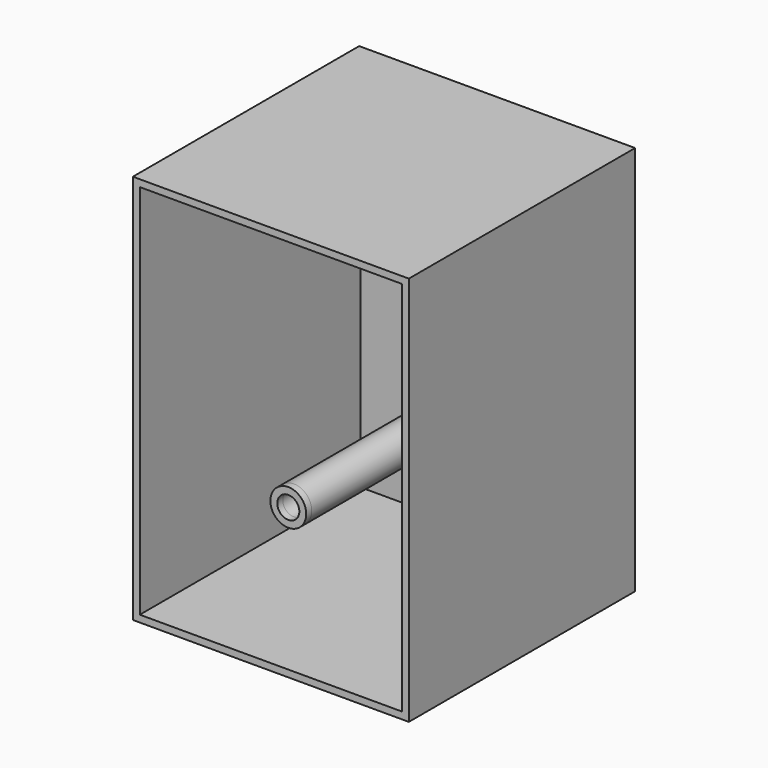
from build123d import *

# Parameters (mm, degrees)
F0_W     = 1000
F0_H     = 1079.8176152468
F1_DEPTH = 1000
F2_R     = 40
F3_DEPTH = 1463.3684158325
F4_DEPTH = 25
F5_DEPTH = 334.466189146
F6_T     = -25
F7_R     = 10


with BuildPart() as f1:
    # F0 (on Front) → F1 (new body)
    with BuildSketch(Plane.XZ):
        with Locations((-87.0127184317, -2.3948438466)):
            Rectangle(F0_W, F0_H)
    extrude(amount=F1_DEPTH)

    # F2 (on face) → F3 (cut)
    with BuildSketch(Plane.XZ.offset(1000)):
        with Locations((-23.8594158151, 0)):
            Circle(F2_R)
    extrude(amount=-F3_DEPTH, mode=Mode.SUBTRACT)

    # F4 (add): a face of the model
    f4_faces = [f1.faces().sort_by_distance(p)[0] for p in [
        (-87.3080717633, -1000, -2.4060439751),
    ]]
    extrude(f4_faces, amount=F4_DEPTH)

    # F5 (add): a face of the model
    f5_faces = [f1.faces().sort_by_distance(p)[0] for p in [
        (-87.0127184317, -512.5, 537.5139637768),
    ]]
    extrude(f5_faces, amount=F5_DEPTH)

    # F6
    f6_openings = [f1.faces().sort_by_distance(p)[0] for p in [
        (-87.237974, -1025, 165.426197),
    ]]
    offset(amount=F6_T, openings=f6_openings)

    # F7
    f7_edges = [f1.edges().sort_by_distance(p)[0] for p in [
        (-88.859416, -25, 0),
    ]]
    fillet(f7_edges, radius=F7_R)


solid = f1.part
